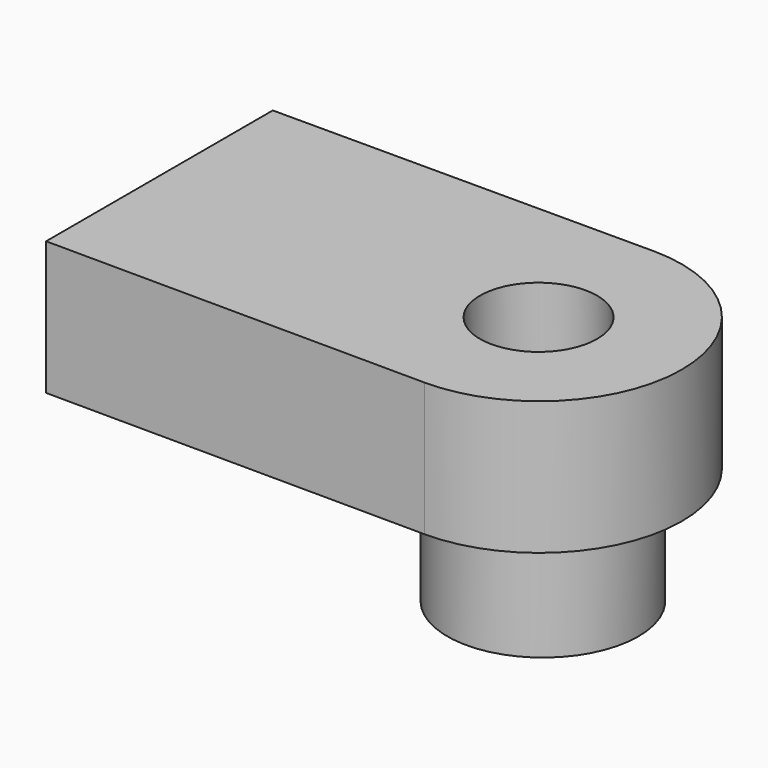
from build123d import *

# Parameters (mm, degrees)
F0_R            = 2.3749
F1_DEPTH        = 6.6548
F2_R            = 4.7625
F3_DEPTH        = 5.842
F5_DEPTH        = 5.842
F5_COPIES_COUNT = 8
F7_R            = 2.921
F8_DEPTH        = 22.225


# Not quite as in the source:
# - a pattern or mirror of a feature is missing from the dataset's text; its kind, count and spacing are read off the source's solid


with BuildPart() as f1:
    # F0 (on Top) → F1 (new body)
    with BuildSketch(Plane.XY):
        with BuildLine():
            ThreePointArc((-0.1195971757, -7.2384254858), (7.0293678249, -0.1863217508), (0, 6.985))
            Line((0, 6.985), (-19.05, 6.985))
            Line((-19.05, 6.985), (-19.05, 0))
            Line((-19.05, 0), (-19.05, -7.1393631719))
            Line((-19.05, -7.1393631719), (-0.1195971757, -7.2384254858))
        make_face()
        with Locations((-0.0823807711, -0.1265228614)):
            Circle(F0_R, mode=Mode.SUBTRACT)
    extrude(amount=F1_DEPTH)

    # F2 (on Top) → F3 (join)
    with BuildSketch(Plane.XY):
        Circle(F2_R)
    extrude(amount=-F3_DEPTH)

    # F4 (on face) → F5 (cut)
    with BuildSketch(Plane(origin=(0, 0, -5.842), x_dir=(1, 0, 0), z_dir=(0, 0, -1))):
        Polygon((0, 1.3200769899), (0, 0), (0, -1.2728312286), (2.831584774, -1.2728312286), (3.7898337469, 0), (2.916136058, 1.3200769899), align=None)
    f5 = extrude(amount=-F5_DEPTH, mode=Mode.SUBTRACT)

    # F5_copies: F5 ×8 about axis
    f5_copies_axis = Axis((0, 0, 0), (0, 0, 1))
    for i in range(1, F5_COPIES_COUNT):
        add(f5.rotate(f5_copies_axis, i * 360 / F5_COPIES_COUNT), mode=Mode.SUBTRACT)

    # F7 (on offset) → F8 (cut)
    with BuildSketch(Plane.XY.offset(25.4)):
        with Locations((-0.0807045596, -0.1689054021)):
            Circle(F7_R)
    extrude(amount=-F8_DEPTH, mode=Mode.SUBTRACT)


solid = f1.part
